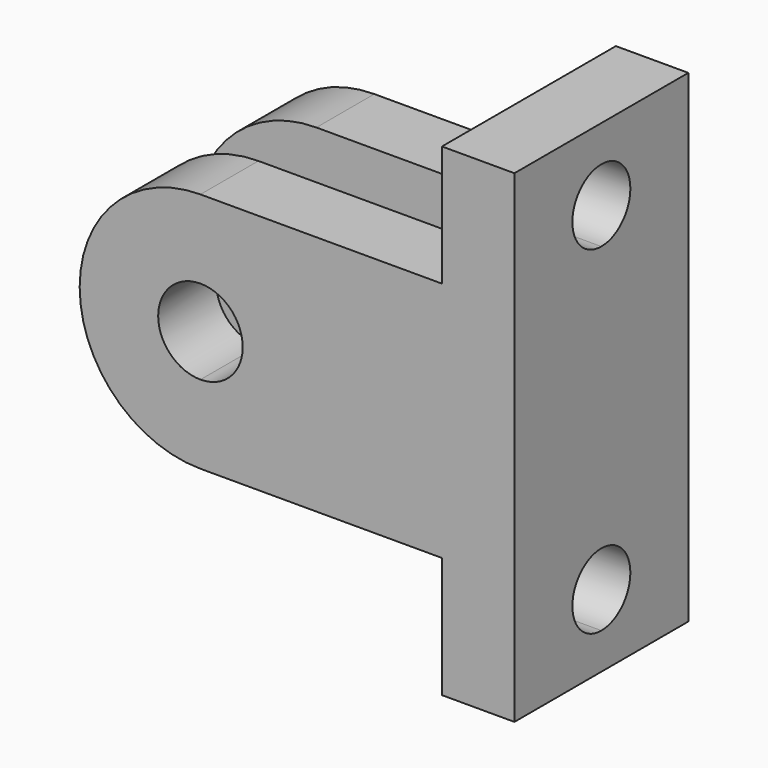
from build123d import *

# Parameters (mm, degrees)
F1_DEPTH = 9
F2_W     = 10
F2_H     = 3
F2_W_2   = 6
F3_DEPTH = 11.5
F5_DEPTH = 3


with BuildPart() as f1:
    # F0 (on Front) → F1 (new body)
    with BuildSketch(Plane.XZ):
        Polygon((-1.5, -10), (1.5, -10), (1.5, 10), (-1.5, 10), (-1.5, 5), (-1.5, 0), (-1.5, -5), align=None)
        with BuildLine():
            ThreePointArc((-11.5, 5), (-16.5, 0), (-11.5, -5))
            Line((-11.5, -5), (-11.5, -1.75))
            ThreePointArc((-11.5, -1.75), (-13.25, 0), (-11.5, 1.75))
            Line((-11.5, 1.75), (-11.5, 5))
        make_face()
        with BuildLine():
            Line((-11.5, -5), (-1.5, -5))
            Line((-1.5, -5), (-1.5, 0))
            Line((-1.5, 0), (-1.5, 5))
            Line((-1.5, 5), (-11.5, 5))
            Line((-11.5, 5), (-11.5, 1.75))
            ThreePointArc((-11.5, 1.75), (-10.2625631329, 1.2374368671), (-9.75, 0))
            ThreePointArc((-9.75, 0), (-10.2625631329, -1.2374368671), (-11.5, -1.75))
            Line((-11.5, -1.75), (-11.5, -5))
        make_face()
    extrude(amount=F1_DEPTH)

    # F2 (on face) → F3 (cut)
    with BuildSketch(Plane(origin=(0, 0, -5), x_dir=(1, 0, 0), z_dir=(0, 0, -1))):
        with Locations((-6.5, 4.5)):
            Rectangle(F2_W, F2_H)
        with Locations((-14.5, 4.5)):
            Rectangle(F2_W_2, F2_H)
    extrude(amount=-F3_DEPTH, mode=Mode.SUBTRACT)

    # F4 (on face) → F5 (cut)
    with BuildSketch(Plane(origin=(-1.5, 0, 0), x_dir=(0, -1, 0), z_dir=(-1, 0, 0))):
        with BuildLine():
            ThreePointArc((4.5, -5.5), (3, -7), (4.5, -8.5))
            Line((4.5, -8.5), (4.5, -5.5))
        make_face()
        with BuildLine():
            Line((4.5, -5.5), (4.5, -8.5))
            ThreePointArc((4.5, -8.5), (5.5606601718, -8.0606601718), (6, -7))
            ThreePointArc((6, -7), (5.5606601718, -5.9393398282), (4.5, -5.5))
        make_face()
        with BuildLine():
            ThreePointArc((4.5, 8.5), (3, 7), (4.5, 5.5))
            Line((4.5, 5.5), (4.5, 8.5))
        make_face()
        with BuildLine():
            Line((4.5, 8.5), (4.5, 5.5))
            ThreePointArc((4.5, 5.5), (5.5606601718, 5.9393398282), (6, 7))
            ThreePointArc((6, 7), (5.5606601718, 8.0606601718), (4.5, 8.5))
        make_face()
    extrude(amount=-F5_DEPTH, mode=Mode.SUBTRACT)


solid = f1.part
